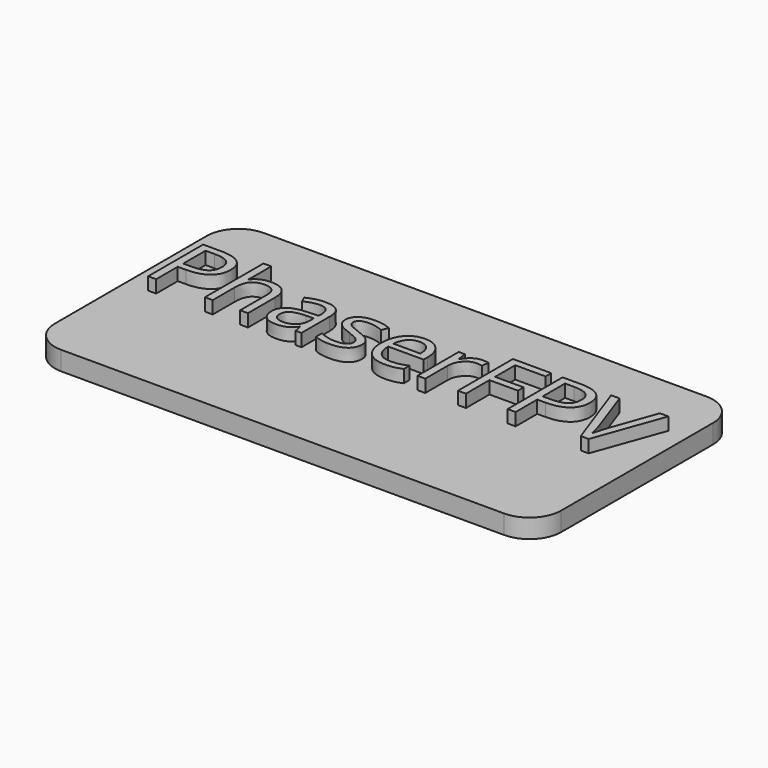
from build123d import *

# Parameters (mm, degrees)
F0_W         = 80
F0_H         = 40
F1_DEPTH     = 3
F2_TEXT_SIZE = 15.210932858
F3_DEPTH     = 2
F4_R         = 5


# Not quite as in the source:
# - Text() gives the source's letters only with a copy of the font that has no kerning and outlines rounded to 1/6400 em; it was checked with that copy


with BuildPart() as f1:
    # F0 (on Top) → F1 (new body)
    with BuildSketch(Plane.XY):
        with Locations((0.1806188375, 17.5696238259)):
            Rectangle(F0_W, F0_H)
    extrude(amount=F1_DEPTH)

    # F2 (on face) → F3 (join)
    with BuildSketch(Plane.XY.offset(3)):
        with Locations((-37.8193811625, 16.6177521681)):
            Text('PhaserFPV', F2_TEXT_SIZE, font='Open Sans', text_align=(TextAlign.LEFT, TextAlign.BOTTOM))
    extrude(amount=F3_DEPTH)

    # F4
    f4_edges = [f1.edges().sort_by_distance(p)[0] for p in [
        (-39.819381, -2.430376, 1.5),
        (40.180619, -2.430376, 1.5),
        (40.180619, 37.569624, 1.5),
        (-39.819381, 37.569624, 1.5),
    ]]
    fillet(f4_edges, radius=F4_R)


solid = f1.part
